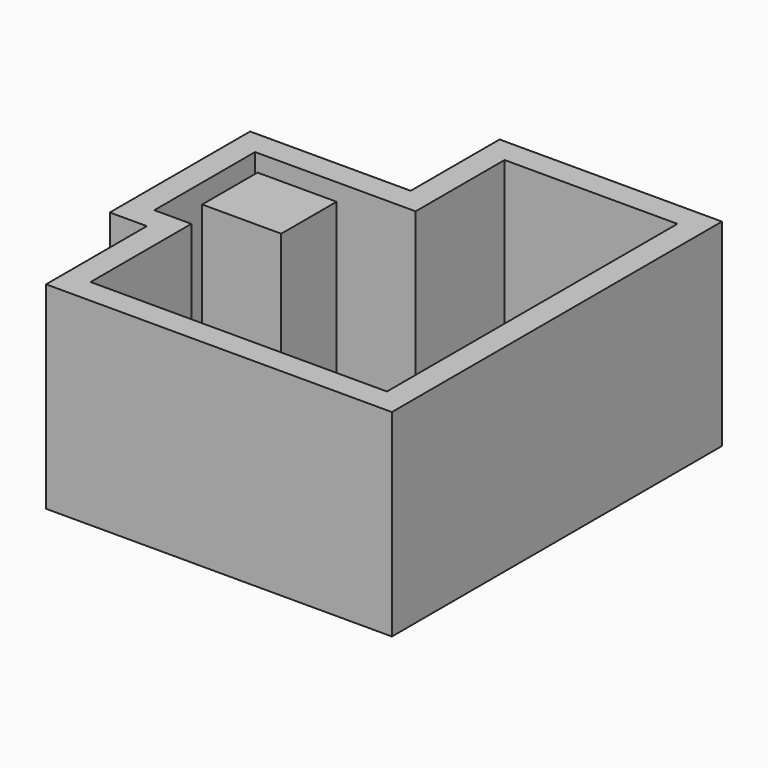
from build123d import *

# Parameters (mm, degrees)
F1_DEPTH       = 75
F2_T           = -0.01
F5_DEPTH       = 10
F6_DEPTH       = 10
F7_DEPTH       = 10
F8_DEPTH       = 10
F9_DEPTH       = 10
F10_DEPTH      = 10
F11_DEPTH      = 10
F12_DEPTH      = 10
F13_DEPTH      = 5
F4_E8_BOTTOM_W = 32
F4_E8_BOTTOM_H = 28
F14_DEPTH      = 0.01
F15_DEPTH      = 68


with BuildPart() as f1:
    # F0 (on Top) → F1 (new body)
    with BuildSketch(Plane.XY):
        Polygon((0, -147), (0, 0), (-70, 0), (-70, -45), (-135, -45), (-135, -96), (-120, -96), (-120, -147), align=None)
    extrude(amount=F1_DEPTH)

    # F2
    f2_openings = [f1.faces().sort_by_distance(p)[0] for p in [
        (-58.321727, -80.461003, 75),
    ]]
    offset(amount=F2_T, openings=f2_openings, kind=Kind.INTERSECTION)

    # F5 (add): a face of the model
    f5_faces = [f1.faces().sort_by_distance(p)[0] for p in [
        (0, -73.5, 37.5),
    ]]
    extrude(f5_faces, amount=F5_DEPTH)

    # F6 (add): a face of the model
    f6_faces = [f1.faces().sort_by_distance(p)[0] for p in [
        (-30, 0, 37.5),
    ]]
    extrude(f6_faces, amount=F6_DEPTH)

    # F7 (add): a face of the model
    f7_faces = [f1.faces().sort_by_distance(p)[0] for p in [
        (-70, -17.5, 37.5),
    ]]
    extrude(f7_faces, amount=F7_DEPTH)

    # F8 (add): a face of the model
    f8_faces = [f1.faces().sort_by_distance(p)[0] for p in [
        (-107.5, -45, 37.5),
    ]]
    extrude(f8_faces, amount=F8_DEPTH)

    # F9 (add): a face of the model
    f9_faces = [f1.faces().sort_by_distance(p)[0] for p in [
        (-135, -65.5, 37.5),
    ]]
    extrude(f9_faces, amount=F9_DEPTH)

    # F10 (add): a face of the model
    f10_faces = [f1.faces().sort_by_distance(p)[0] for p in [
        (-132.5, -96, 37.5),
    ]]
    extrude(f10_faces, amount=F10_DEPTH)

    # F11 (add): a face of the model
    f11_faces = [f1.faces().sort_by_distance(p)[0] for p in [
        (-120, -126.5, 37.5),
    ]]
    extrude(f11_faces, amount=F11_DEPTH)

    # F12 (add): a face of the model
    f12_faces = [f1.faces().sort_by_distance(p)[0] for p in [
        (-60, -147, 37.5),
    ]]
    extrude(f12_faces, amount=F12_DEPTH)

    # F13 (add): a face of the model
    f13_faces = [f1.faces().sort_by_distance(p)[0] for p in [
        (-59.1569047083, -79.5398738455, 0),
    ]]
    extrude(f13_faces, amount=F13_DEPTH)

    # F4_E8_bottom (on explicit) → F14 (join, through all)
    with BuildSketch(Plane(origin=(-134, -45, 0), x_dir=(1, 0, 0), z_dir=(0, 0, -1))):
        with Locations((16, 14)):
            Rectangle(F4_E8_BOTTOM_W, F4_E8_BOTTOM_H)
    extrude(amount=-F14_DEPTH)

    # F4_E8_bottom (on explicit) → F15 (join)
    with BuildSketch(Plane(origin=(-134, -45, 0), x_dir=(1, 0, 0), z_dir=(0, 0, -1))):
        with Locations((16, 14)):
            Rectangle(F4_E8_BOTTOM_W, F4_E8_BOTTOM_H)
    extrude(amount=-F15_DEPTH)


solid = f1.part
